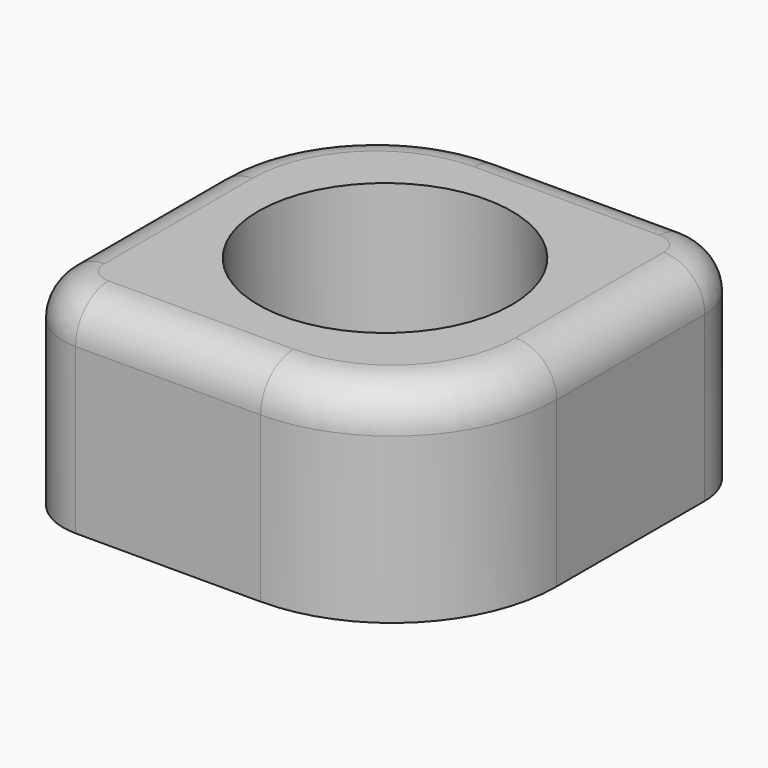
from build123d import *

# Parameters (mm, degrees)
F0_W        = 100
F0_H        = 100
F1_DEPTH    = 50
F2_R        = 10
F3_T1_DEPTH = 150
F3_T4_ANGLE = 90
F3_T6_ANGLE = 90
F4_T1_DEPTH = 87.5
F4_T4_ANGLE = 90
F4_T6_ANGLE = 90
F5_R        = 30.8330010445
F6_DEPTH    = 40


# Not quite as in the source:
# - a fillet or chamfer that OpenCascade refuses, or shapes differently, is made with other operations: its cross-section is extruded or revolved along the edge and cut away or added


with BuildPart() as f1:
    # F0 (on Top) → F1 (new body)
    with BuildSketch(Plane.XY):
        with Locations((-16.9892802835, -14.8166164756)):
            Rectangle(F0_W, F0_H)
    extrude(amount=F1_DEPTH)

    # F2
    f2_edges = [f1.edges().sort_by_distance(p)[0] for p in [
        (-16.98928, -64.816616, 50),
        (33.01072, -14.816616, 50),
        (-16.98928, 35.183384, 50),
        (-66.98928, -14.816616, 50),
    ]]
    fillet(f2_edges, radius=F2_R)

    # F3: fillet of radius 40 on 2 edges, made by hand

    # F3_s2 → F3_t1 (cut)
    with BuildSketch(Plane.XY.offset(-100)):
        with BuildLine():
            ThreePointArc((33.0107197165, -24.8166164756), (21.294990964, -53.100887723), (-6.9892802835, -64.8166164756))
            Line((-6.9892802835, -64.8166164756), (33.0107197165, -64.8166164756))
            Line((33.0107197165, -64.8166164756), (33.0107197165, -24.8166164756))
        make_face()
        with BuildLine():
            ThreePointArc((-26.9892802835, 35.1833835244), (-55.2735515309, 23.4676547719), (-66.9892802835, -4.8166164756))
            Line((-66.9892802835, -4.8166164756), (-66.9892802835, 35.1833835244))
            Line((-66.9892802835, 35.1833835244), (-26.9892802835, 35.1833835244))
        make_face()
    extrude(amount=F3_T1_DEPTH, mode=Mode.SUBTRACT)

    # F3_s3 → F3_t4 (revolve, cut)
    with BuildSketch(Plane.YZ.offset(-26.9892802835)):
        with BuildLine():
            ThreePointArc((25.1833835244, 50), (32.2544513363, 47.0710678119), (35.1833835244, 40))
            Line((35.1833835244, 40), (35.1833835244, 50))
            Line((35.1833835244, 50), (25.1833835244, 50))
        make_face()
    revolve(axis=Axis((-26.9892802835, -4.8166164756, 50), (0, 0, 1)), revolution_arc=F3_T4_ANGLE, mode=Mode.SUBTRACT)

    # F3_s5 → F3_t6 (revolve, cut)
    with BuildSketch(Plane.YZ.offset(-6.9892802835)):
        with BuildLine():
            ThreePointArc((-54.8166164756, 50), (-61.8876842874, 47.0710678119), (-64.8166164756, 40))
            Line((-64.8166164756, 40), (-64.8166164756, 50))
            Line((-64.8166164756, 50), (-54.8166164756, 50))
        make_face()
    revolve(axis=Axis((-6.9892802835, -24.8166164756, 50), (0, 0, 1)), revolution_arc=F3_T6_ANGLE, mode=Mode.SUBTRACT)

    # F4: fillet of radius 15 on 2 edges, made by hand

    # F4_s2 → F4_t1 (cut)
    with BuildSketch(Plane.XY.offset(-37.5)):
        with BuildLine():
            ThreePointArc((33.0107197165, 20.1833835244), (28.6173214343, 30.7899852422), (18.0107197165, 35.1833835244))
            Line((18.0107197165, 35.1833835244), (33.0107197165, 35.1833835244))
            Line((33.0107197165, 35.1833835244), (33.0107197165, 20.1833835244))
        make_face()
        with BuildLine():
            ThreePointArc((-51.9892802835, -64.8166164756), (-62.5958820012, -60.4232181934), (-66.9892802835, -49.8166164756))
            Line((-66.9892802835, -49.8166164756), (-66.9892802835, -64.8166164756))
            Line((-66.9892802835, -64.8166164756), (-51.9892802835, -64.8166164756))
        make_face()
    extrude(amount=F4_T1_DEPTH, mode=Mode.SUBTRACT)

    # F4_s3 → F4_t4 (revolve, cut)
    with BuildSketch(Plane.XZ.offset(49.8166164756)):
        with BuildLine():
            ThreePointArc((-56.9892802835, 50), (-64.0603480953, 47.0710678119), (-66.9892802835, 40))
            Line((-66.9892802835, 40), (-66.9892802835, 50))
            Line((-66.9892802835, 50), (-56.9892802835, 50))
        make_face()
    revolve(axis=Axis((-51.9892802835, -49.8166164756, 50), (0, 0, 1)), revolution_arc=F4_T4_ANGLE, mode=Mode.SUBTRACT)

    # F4_s5 → F4_t6 (revolve, cut)
    with BuildSketch(Plane.XZ.offset(-20.1833835244)):
        with BuildLine():
            ThreePointArc((23.0107197165, 50), (30.0817875284, 47.0710678119), (33.0107197165, 40))
            Line((33.0107197165, 40), (33.0107197165, 50))
            Line((33.0107197165, 50), (23.0107197165, 50))
        make_face()
    revolve(axis=Axis((18.0107197165, 20.1833835244, 50), (0, 0, 1)), revolution_arc=F4_T6_ANGLE, mode=Mode.SUBTRACT)

    # F5 (on face) → F6 (cut)
    with BuildSketch(Plane.XY.offset(50)):
        with Locations((-16.8512575328, -14.6785899997)):
            Circle(F5_R)
    extrude(amount=-F6_DEPTH, mode=Mode.SUBTRACT)


solid = f1.part
